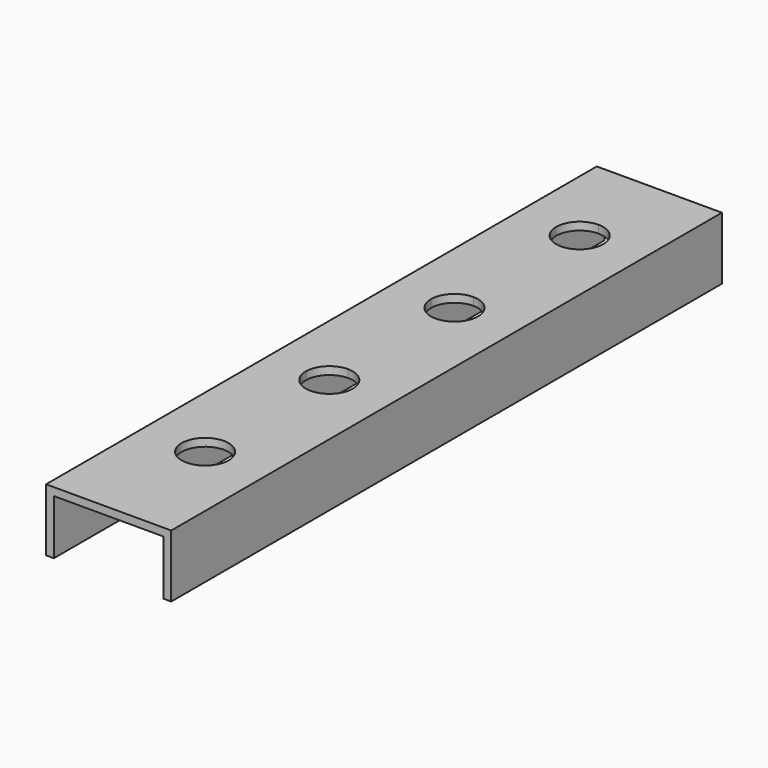
from build123d import *

# Parameters (mm, degrees)
F1_DEPTH = 279.4
F3_DEPTH = 25.401
F5_D     = 19.05


# Not quite as in the source:
# - a feature names something its author has since deleted; it is built from what else it names


with BuildPart() as f1:
    # F0 (on Front) → F1 (new body)
    with BuildSketch(Plane.XZ):
        Polygon((25.4, -12.7), (25.4, 12.7), (-25.4, 12.7), (-25.4, -12.7), (-22.225, -12.7), (-22.225, 9.525), (22.225, 9.525), (22.225, -12.7), align=None)
    extrude(amount=F1_DEPTH)

    # F2 (on face) → F3 (cut, through all)
    with BuildSketch(Plane.XY.offset(12.7)):
        with BuildLine():
            Line((0, -40.4343813046), (9.525, -40.4343813046))
            ThreePointArc((9.525, -40.4343813046), (6.7351920908, -33.6991892138), (0, -30.9093813046))
            Line((0, -30.9093813046), (0, -40.4343813046))
        make_face()
        with BuildLine():
            ThreePointArc((0, -30.9093813046), (-6.7351920908, -33.6991892138), (-9.525, -40.4343813046))
            Line((-9.525, -40.4343813046), (0, -40.4343813046))
            Line((0, -40.4343813046), (0, -30.9093813046))
        make_face()
        with BuildLine():
            Line((0, -40.4343813046), (-9.525, -40.4343813046))
            ThreePointArc((-9.525, -40.4343813046), (-6.7351920908, -47.1695733954), (0, -49.9593813046))
            Line((0, -49.9593813046), (0, -40.4343813046))
        make_face()
        with BuildLine():
            Line((0, -103.9343813046), (9.525, -103.9343813046))
            ThreePointArc((9.525, -103.9343813046), (6.7351920908, -97.1991892138), (0, -94.4093813046))
            Line((0, -94.4093813046), (0, -103.9343813046))
        make_face()
        with BuildLine():
            ThreePointArc((0, -94.4093813046), (-6.7351920908, -97.1991892138), (-9.525, -103.9343813046))
            Line((-9.525, -103.9343813046), (0, -103.9343813046))
            Line((0, -103.9343813046), (0, -94.4093813046))
        make_face()
        with BuildLine():
            ThreePointArc((0, -113.4593813046), (6.7351920908, -110.6695733954), (9.525, -103.9343813046))
            Line((9.525, -103.9343813046), (0, -103.9343813046))
            Line((0, -103.9343813046), (0, -113.4593813046))
        make_face()
        with BuildLine():
            Line((0, -103.9343813046), (-9.525, -103.9343813046))
            ThreePointArc((-9.525, -103.9343813046), (-6.7351920908, -110.6695733954), (0, -113.4593813046))
            Line((0, -113.4593813046), (0, -103.9343813046))
        make_face()
        with BuildLine():
            Line((0, -167.4343813046), (9.525, -167.4343813046))
            ThreePointArc((9.525, -167.4343813046), (6.7351920908, -160.6991892138), (0, -157.9093813046))
            Line((0, -157.9093813046), (0, -167.4343813046))
        make_face()
        with BuildLine():
            ThreePointArc((0, -157.9093813046), (-6.7351920908, -160.6991892138), (-9.525, -167.4343813046))
            Line((-9.525, -167.4343813046), (0, -167.4343813046))
            Line((0, -167.4343813046), (0, -157.9093813046))
        make_face()
        with BuildLine():
            Line((0, -167.4343813046), (0, -176.9593813046))
            ThreePointArc((0, -176.9593813046), (6.7351920908, -174.1695733954), (9.525, -167.4343813046))
            Line((9.525, -167.4343813046), (0, -167.4343813046))
        make_face()
        with BuildLine():
            ThreePointArc((-9.525, -167.4343813046), (-6.7351920908, -174.1695733954), (0, -176.9593813046))
            Line((0, -176.9593813046), (0, -167.4343813046))
            Line((0, -167.4343813046), (-9.525, -167.4343813046))
        make_face()
        with BuildLine():
            Line((0, -220.9396968842), (0, -230.4646968842))
            Line((0, -230.4646968842), (9.525, -230.4646968842))
            ThreePointArc((9.525, -230.4646968842), (6.7351920908, -223.7295047934), (0, -220.9396968842))
        make_face()
        with BuildLine():
            Line((-9.525, -230.4646968842), (0, -230.4646968842))
            Line((0, -230.4646968842), (0, -220.9396968842))
            ThreePointArc((0, -220.9396968842), (-6.7351920908, -223.7295047934), (-9.525, -230.4646968842))
        make_face()
        with BuildLine():
            ThreePointArc((0, -49.9593813046), (6.7351920908, -47.1695733954), (9.525, -40.4343813046))
            Line((9.525, -40.4343813046), (0, -40.4343813046))
            Line((0, -40.4343813046), (0, -49.9593813046))
        make_face()
    extrude(amount=-F3_DEPTH, mode=Mode.SUBTRACT)

    # F5 (through all)
    with Locations(Plane.XY.offset(12.7)):
        with Locations((0, -230.4646968842)):
            Hole(F5_D / 2)


solid = f1.part
